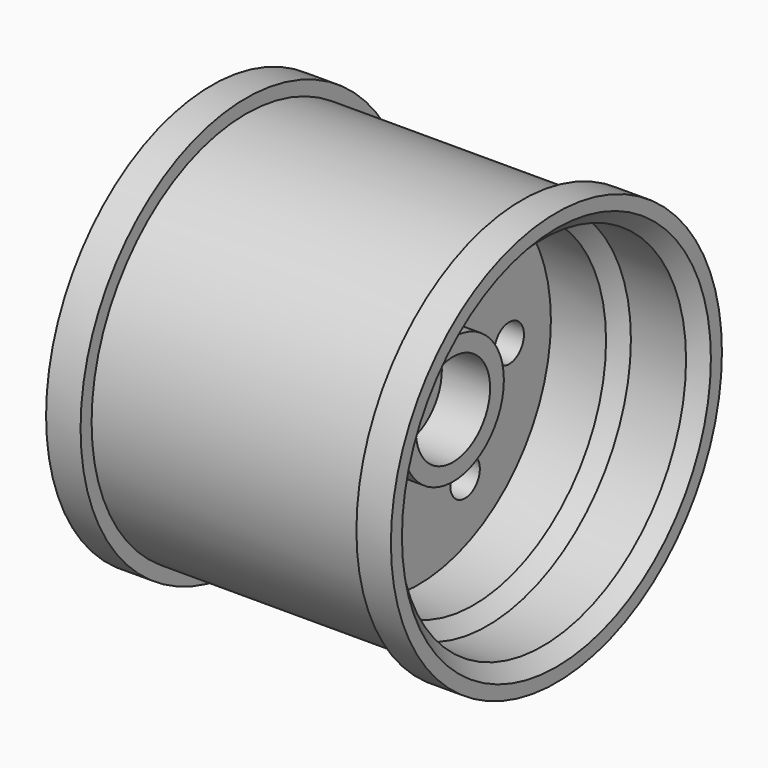
from build123d import *

# Parameters (mm, degrees)
F0_R     = 15
F0_R_2   = 14
F0_R_3   = 13
F1_DEPTH = 12.5
F0_R_4   = 12
F2_DEPTH = 7.5
F0_R_5   = 1.340335668
F0_R_6   = 4.6127208632
F3_DEPTH = 2.5
F0_R_7   = 3.3654242234
F4_DEPTH = 5
F0_R_8   = 1.513947391
F5_DEPTH = 1.5
F6_DEPTH = 10
F7_SIZE  = 0.99999
F8_SIZE  = 1


# Not quite as in the source:
# - a fillet or chamfer is up to 0.001 mm smaller than in the source, because OpenCascade refuses the exact size


with BuildPart() as f1:
    # F0 (on Right) → F1 (new body, symmetric)
    with BuildSketch(Plane.YZ):
        Circle(F0_R)
        Circle(F0_R_2, mode=Mode.SUBTRACT)
        Circle(F0_R_2)
        Circle(F0_R_3, mode=Mode.SUBTRACT)
    extrude(amount=F1_DEPTH, both=True)

    # F0 (on Right) → F6 (cut, symmetric)
    with BuildSketch(Plane.YZ):
        Circle(F0_R)
        Circle(F0_R_2, mode=Mode.SUBTRACT)
    extrude(amount=F6_DEPTH, both=True, mode=Mode.SUBTRACT)

    # F8
    f8_edges = [f1.edges().sort_by_distance(p)[0] for p in [
        (-12.5, -13, 0),
        (12.5, -13, 0),
    ]]
    chamfer(f8_edges, length=F8_SIZE)


with BuildPart() as f2:
    # F0 (on Right) → F2 (new body, symmetric)
    with BuildSketch(Plane.YZ):
        Circle(F0_R_3)
        Circle(F0_R_4, mode=Mode.SUBTRACT)
    extrude(amount=F2_DEPTH, both=True)

    # F0 (on Right) → F3 (join)
    with BuildSketch(Plane.YZ):
        Circle(F0_R_4)
        with Locations((-3.7932281848, -6.8703168072)):
            Circle(F0_R_5, mode=Mode.SUBTRACT)
        with Locations((4.2197729637, -6.8601384378)):
            Circle(F0_R_5, mode=Mode.SUBTRACT)
        with Locations((-7.8085434855, 0.0640565633)):
            Circle(F0_R_5, mode=Mode.SUBTRACT)
        with Locations((-3.8108576376, 7.0086083031)):
            Circle(F0_R_5, mode=Mode.SUBTRACT)
        Circle(F0_R_6, mode=Mode.SUBTRACT)
        with Locations((4.2021435108, 7.0187866725)):
            Circle(F0_R_5, mode=Mode.SUBTRACT)
        with Locations((8.2174588115, 0.084413302)):
            Circle(F0_R_5, mode=Mode.SUBTRACT)
    extrude(amount=F3_DEPTH)

    # F0 (on Right) → F4 (join, symmetric)
    with BuildSketch(Plane.YZ):
        Circle(F0_R_6)
        Circle(F0_R_7, mode=Mode.SUBTRACT)
    extrude(amount=F4_DEPTH, both=True)

    # F0 (on Right) → F5 (join, symmetric)
    with BuildSketch(Plane.YZ):
        Circle(F0_R_7)
        Circle(F0_R_8, mode=Mode.SUBTRACT)
    extrude(amount=F5_DEPTH, both=True)

    # F7 (size 1 in the source; OpenCascade refuses exactly that, so slightly less here)
    f7_edges = [f2.edges().sort_by_distance(p)[0] for p in [
        (7.5, -12, 0),
        (-7.5, -12, 0),
    ]]
    chamfer(f7_edges, length=F7_SIZE)


solid = Compound([f1.part, f2.part])
